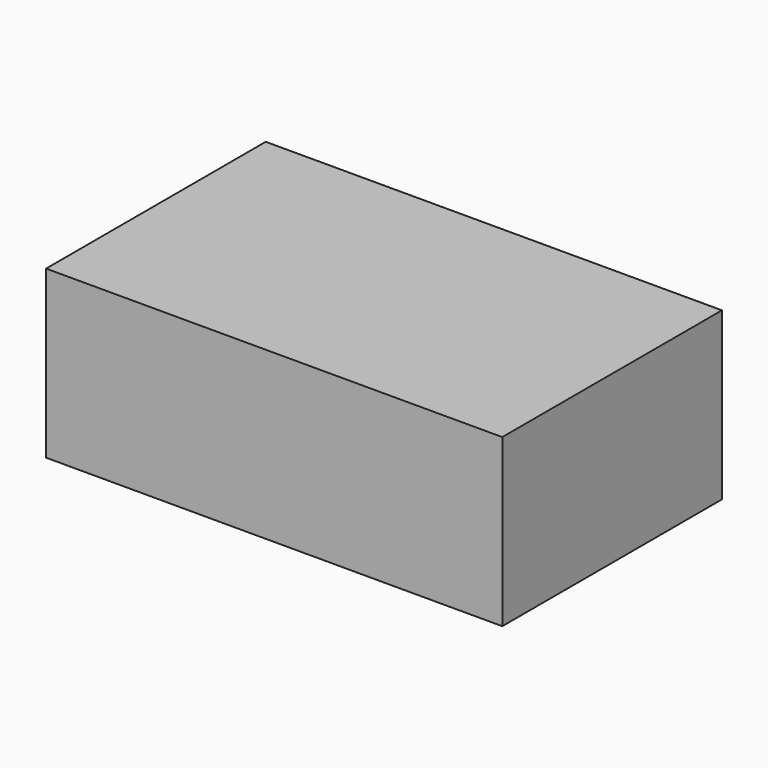
from build123d import *

# Parameters (mm, degrees)
F0_W     = 69.5927813649
F0_H     = 41.8875440955
F1_DEPTH = 25.4


# Not quite as in the source:
# - a feature of the source that left no trace in its solid (it failed there, or was rolled back) is left out


with BuildPart() as f1:
    # F0 (on Top) → F1 (new body)
    with BuildSketch(Plane.XY):
        with Locations((-34.7963906825, -6.5461024642)):
            Rectangle(F0_W, F0_H)
    extrude(amount=F1_DEPTH)


solid = f1.part
